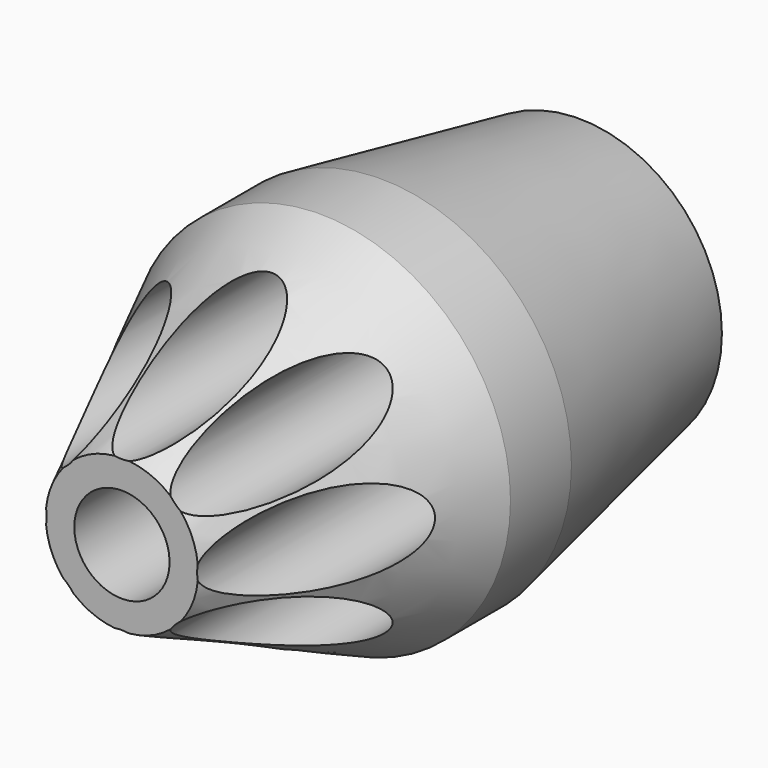
from build123d import *

# Parameters (mm, degrees)
F0_R      = 12.7
F1_DEPTH  = 38.1
F3_D      = 11.90752
F3_DEPTH  = 15.4214285714
F3_TIP    = 3.5773799191
F5_D      = 6.35
F7_D      = 5.842
F7_DEPTH  = 25.4
F7_TIP    = 1.7551138682
F12_SIZE2 = 3.175
F12_SIZE  = 16.51


# Not quite as in the source:
# - a fillet or chamfer that OpenCascade refuses, or shapes differently, is made with other operations: its cross-section is extruded or revolved along the edge and cut away or added


with BuildPart() as f1:
    # F0 (on Front) → F1 (new body)
    with BuildSketch(Plane.XZ):
        Circle(F0_R)
    extrude(amount=F1_DEPTH)

    # F3
    with Locations(Plane(origin=(0, 0, 0), x_dir=(-1, 0, 0), z_dir=(0, 1, 0))):
        with Locations((0, 0)):
            Hole(F3_D / 2, depth=F3_DEPTH)
            with Locations((0, 0, -(F3_DEPTH + F3_TIP / 2))):  # 118° drill point
                Cone(0, F3_D / 2, F3_TIP, mode=Mode.SUBTRACT)

    # F5 (through all)
    with Locations(Plane.XZ.offset(38.1)):
        with Locations((0, 0)):
            Hole(F5_D / 2)

    # F7
    with Locations(Plane.XZ.offset(38.1)):
        with Locations((0, 7.9375), (-5.6126600757, 5.6126600757), (-7.9375, 0), (-5.6126600757, -5.6126600757), (0, -7.9375), (5.6126600757, -5.6126600757), (7.9375, 0), (5.6126600757, 5.6126600757)):
            Hole(F7_D / 2, depth=F7_DEPTH)
            with Locations((0, 0, -(F7_DEPTH + F7_TIP / 2))):  # 118° drill point
                Cone(0, F7_D / 2, F7_TIP, mode=Mode.SUBTRACT)

    # F11: chamfer of 7.62 x 16.51 on 1 edges, made by hand

    # F11_s1 → F11_t2 (revolve, cut)
    with BuildSketch(Plane.XY):
        Polygon((12.7, -21.59), (5.08, -38.1), (12.7, -38.1), align=None)
    revolve(axis=Axis((0, -38.1, 0), (0, -1, 0)), mode=Mode.SUBTRACT)

    # F12
    f12_edges = [f1.edges().sort_by_distance(p)[0] for p in [
        (-12.7, 0, 0),
    ]]
    f12_side = f1.faces().sort_by_distance((-12.7, -10.795, 0))[0]
    chamfer(f12_edges, length=F12_SIZE, length2=F12_SIZE2, reference=f12_side)


solid = f1.part
